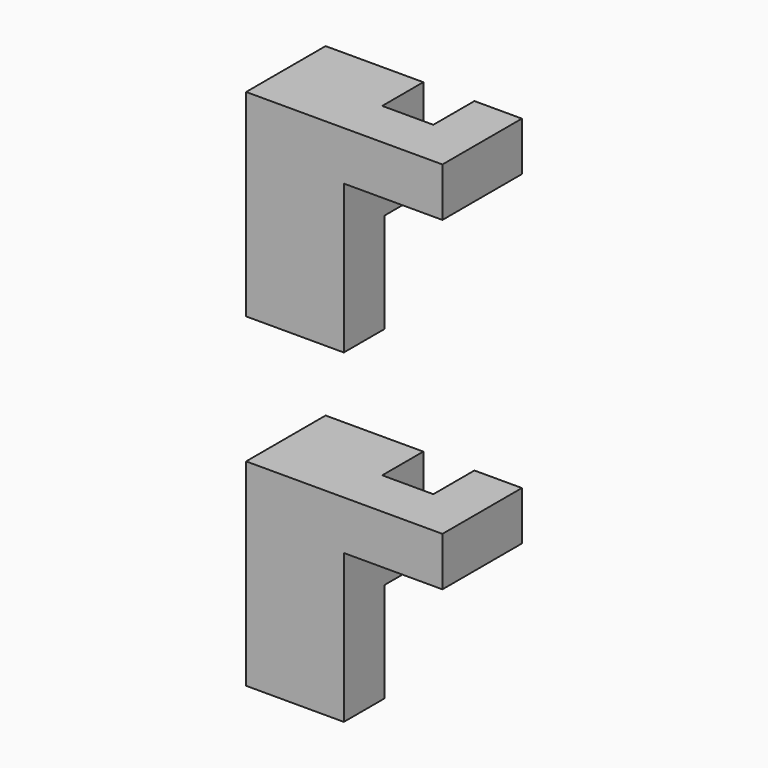
from build123d import *

# Parameters (mm, degrees)
F0_W     = 15.81
F0_H     = 15.81
F1_DEPTH = 16.07
F3_DEPTH = 8.27
F5_DEPTH = 7.68
F6_W     = 15.81
F6_H     = 16.16
F7_DEPTH = 8.26
F9_DEPTH = 7.89


with BuildPart() as f1:
    # F0 (on Front) → F1 (new body)
    with BuildSketch(Plane.XZ):
        Rectangle(F0_W, F0_H)
    extrude(amount=-F1_DEPTH)

    # F2 (on face) → F3 (join)
    with BuildSketch(Plane.YZ.offset(7.905)):
        Polygon((7.76, 7.905), (0, 7.905), (0, 0.145), (0, 0), align=None)
    extrude(amount=F3_DEPTH)

    # F4 (on face) → F5 (join)
    with BuildSketch(Plane.YZ.offset(16.175)):
        Polygon((0, 0), (7.76, 7.905), (0, 7.905), align=None)
        Polygon((16.07, 0), (16.07, 7.905), (7.76, 7.905), (0, 0), align=None)
    extrude(amount=F5_DEPTH)

    # F6 (on face) → F7 (join)
    with BuildSketch(Plane.XZ):
        with Locations((0, -15.985)):
            Rectangle(F6_W, F6_H)
    extrude(amount=-F7_DEPTH)

    # F8 (on face) → F9 (join)
    with BuildSketch(Plane(origin=(-7.905, 0, 0), x_dir=(0, -1, 0), z_dir=(-1, 0, 0))):
        Polygon((-15.56, -24.065), (-8.26, -24.065), (-8.26, -7.905), (-15.56, -16.765), align=None)
    extrude(amount=-F9_DEPTH)


with BuildPart() as f10_1:
    # F10: copy of F1
    add(f1.part.moved(Location((0, 0, 52.61464))))


solid = Compound([f1.part, f10_1.part])
